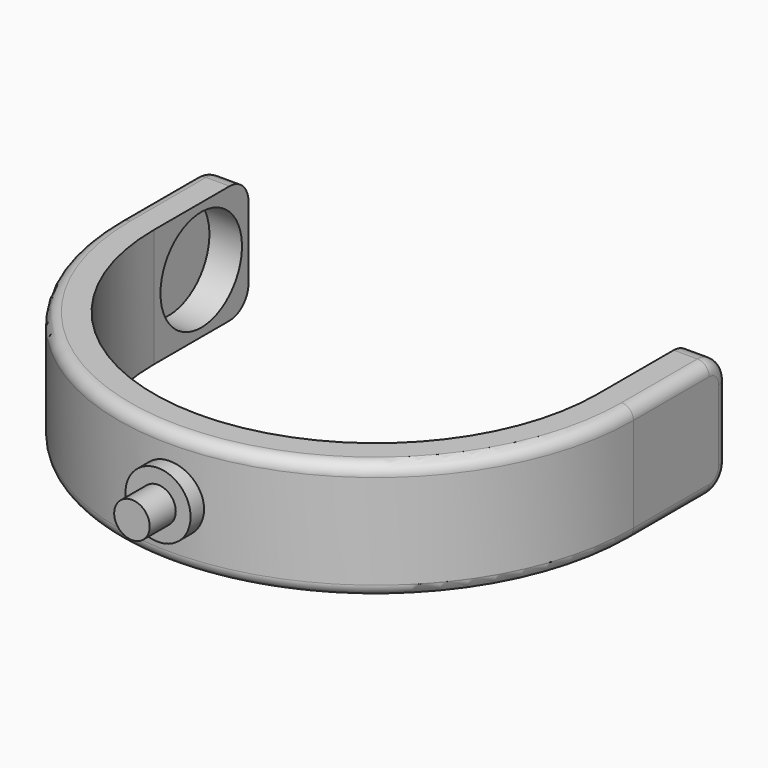
from build123d import *

# Parameters (mm, degrees)
F0_W          = 7.62
F0_H          = 25.4
F1_DEPTH      = 25.4
F5_R          = 10.922
F6_DEPTH      = 6.985
F4_R          = 6.985
F4_R_2        = 3.81
F7_DEPTH      = 3.175
F7_DEPTH_BACK = 3.175
F8_DEPTH      = 10.16
F8_DEPTH_BACK = 3.175
F9_R          = 5.08
F10_R         = 2.54


# Not quite as in the source:
# - a pattern or mirror of a feature is missing from the dataset's text; its kind, count and spacing are read off the source's solid


with BuildPart() as f1:
    # F0 (on Top) → F1 (new body)
    with BuildSketch(Plane.XY):
        with BuildLine():
            Line((55.245, 0), (47.625, 0))
            ThreePointArc((47.625, 0), (0, -47.625), (-47.625, 0))
            Line((-47.625, 0), (-55.245, 0))
            ThreePointArc((-55.245, 0), (0, -55.245), (55.245, 0))
        make_face()
        with Locations((51.435, 12.7)):
            Rectangle(F0_W, F0_H)
        with Locations((-51.435, 12.7)):
            Rectangle(F0_W, F0_H)
    extrude(amount=F1_DEPTH)

    # F5 (on face) → F6 (cut)
    with BuildSketch(Plane(origin=(47.625, 0, 0), x_dir=(0, -1, 0), z_dir=(-1, 0, 0))):
        with Locations((-12.7, 12.7)):
            Circle(F5_R)
    f6 = extrude(amount=-F6_DEPTH, mode=Mode.SUBTRACT)

    # F6_copies: F6 across plane
    add(f6.mirror(Plane(origin=(0, 0, 0), x_dir=(0, 0, -1), z_dir=(-1, 0, 0))), mode=Mode.SUBTRACT)

    # F4 (on plane+point) → F7 (join, two sides)
    with BuildSketch(Plane.XZ.offset(55.245)) as f7_sk:
        with Locations((0, 12.7)):
            Circle(F4_R)
        with Locations((0, 12.7)):
            Circle(F4_R_2, mode=Mode.SUBTRACT)
    extrude(amount=F7_DEPTH)
    extrude(f7_sk.sketch, amount=-F7_DEPTH_BACK)

    # F4 (on plane+point) → F8 (join, two sides)
    with BuildSketch(Plane.XZ.offset(55.245)) as f8_sk:
        with Locations((0, 12.7)):
            Circle(F4_R_2)
    extrude(amount=F8_DEPTH)
    extrude(f8_sk.sketch, amount=-F8_DEPTH_BACK)

    # F9
    f9_edges = [f1.edges().sort_by_distance(p)[0] for p in [
        (-51.435, 25.4, 0),
        (-51.435, 25.4, 25.4),
        (51.435, 25.4, 25.4),
        (51.435, 25.4, 0),
    ]]
    fillet(f9_edges, radius=F9_R)

    # F10
    f10_edges = [f1.edges().sort_by_distance(p)[0] for p in [
        (0, -55.245, 0),
        (55.245, 25.4, 12.7),
        (55.245, 23.912102, 1.487898),
        (55.245, 23.912102, 23.912102),
        (-55.245, 10.16, 0),
        (55.245, 10.16, 0),
        (-55.245, 10.16, 25.4),
        (0, -55.245, 25.4),
        (55.245, 10.16, 25.4),
        (-55.245, 23.912102, 1.487898),
        (-55.245, 25.4, 12.7),
        (-55.245, 23.912102, 23.912102),
    ]]
    fillet(f10_edges, radius=F10_R)


solid = f1.part
